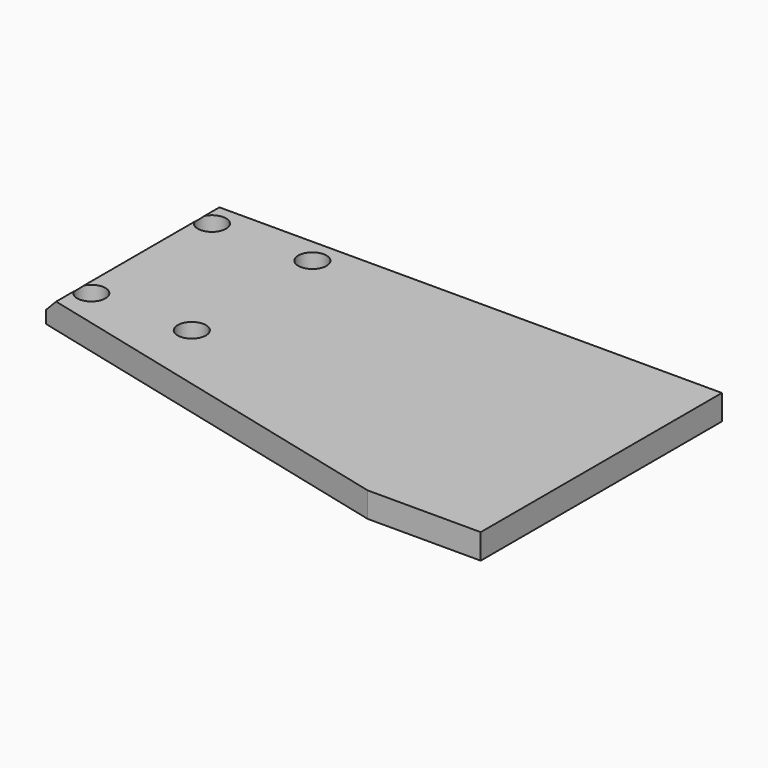
from build123d import *

# Parameters (mm, degrees)
F0_R        = 3.5687
F1_DEPTH    = 6.35
F2_T1_DEPTH = 67.1301869736


# Not quite as in the source:
# - a fillet or chamfer that OpenCascade refuses, or shapes differently, is made with other operations: its cross-section is extruded or revolved along the edge and cut away or added


with BuildPart() as f1:
    # F0 (on Top) → F1 (new body)
    with BuildSketch(Plane.XY):
        Polygon((130.175, 0), (0, 0), (0, -50.8), (101.6, -76.2), (130.175, -76.2), align=None)
        with Locations((6.35, -44.45)):
            Circle(F0_R, mode=Mode.SUBTRACT)
        with Locations((31.75, -44.45)):
            Circle(F0_R, mode=Mode.SUBTRACT)
        with Locations((6.35, -6.35)):
            Circle(F0_R, mode=Mode.SUBTRACT)
        with Locations((31.75, -6.35)):
            Circle(F0_R, mode=Mode.SUBTRACT)
    extrude(amount=F1_DEPTH)

    # F2: chamfer of 3.175 on 1 edges, made by hand

    # F2_s2 → F2_t1 (cut)
    with BuildSketch(Plane.XZ.offset(-8.1650934868)):
        Polygon((0, 3.175), (3.175, 6.35), (0, 6.35), align=None)
    extrude(amount=F2_T1_DEPTH, mode=Mode.SUBTRACT)


solid = f1.part
